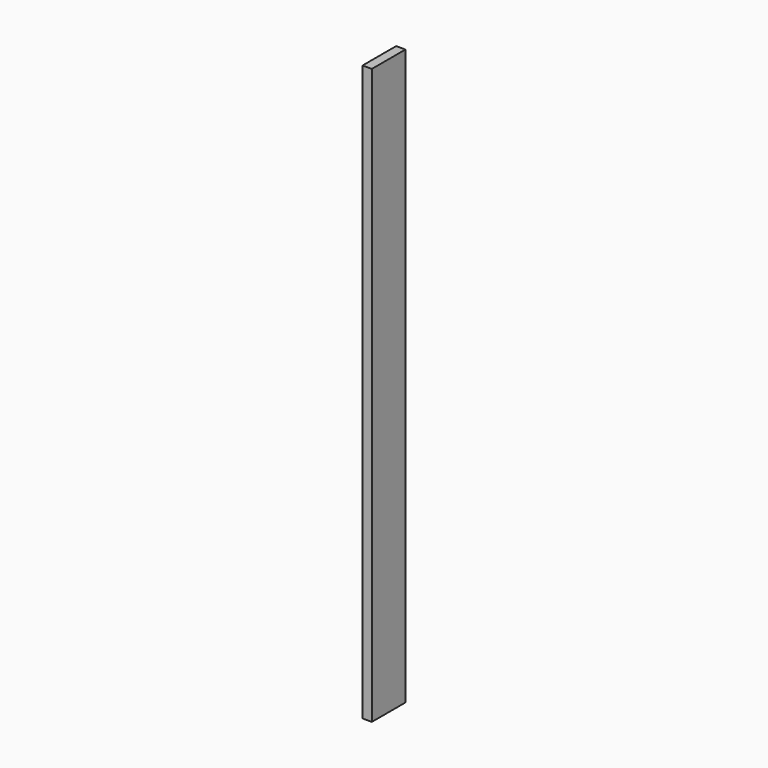
from build123d import *

# Parameters (mm, degrees)
F1_W     = 21
F1_H     = 95
F2_DEPTH = 1300


with BuildPart() as f2:
    # F1 (on Top) → F2 (new body)
    with BuildSketch(Plane.XY):
        with Locations((10.5, 47.5)):
            Rectangle(F1_W, F1_H)
    extrude(amount=F2_DEPTH)


solid = f2.part
